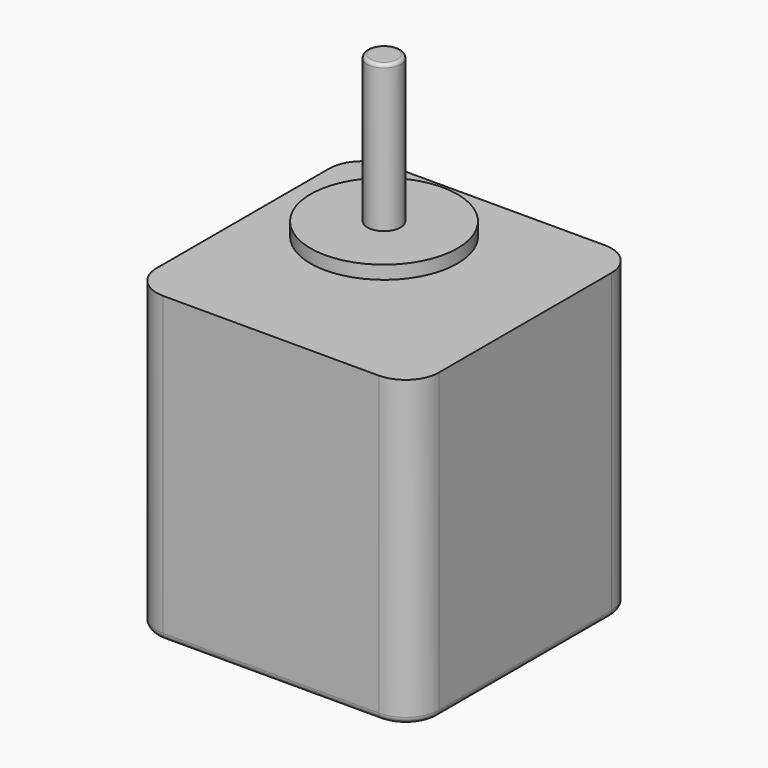
from build123d import *

# Parameters (mm, degrees)
F1_W     = 42.3
F1_H     = 42.3
F1_R     = 1.5
F1_R_2   = 11
F1_R_3   = 2.5
F2_DEPTH = 45.5
F3_START = 50
F3_DEPTH = 2
F4_START = 52
F4_DEPTH = 22
F5_R     = 0.5
F6_R     = 5
F7_R     = 1


with BuildPart() as f2:
    # F1 (on Top) → F2 (new body)
    with BuildSketch(Plane.XY):
        Rectangle(F1_W, F1_H)
        with Locations((-15.5, -15.5)):
            Circle(F1_R, mode=Mode.SUBTRACT)
        with Locations((15.5, -15.5)):
            Circle(F1_R, mode=Mode.SUBTRACT)
        with Locations((-15.5, 15.5)):
            Circle(F1_R, mode=Mode.SUBTRACT)
        Circle(F1_R_2, mode=Mode.SUBTRACT)
        with Locations((15.5, 15.5)):
            Circle(F1_R, mode=Mode.SUBTRACT)
        Circle(F1_R_2)
        Circle(F1_R_3, mode=Mode.SUBTRACT)
        Circle(F1_R_3)
        with Locations((-15.5, 15.5)):
            Circle(F1_R)
        with Locations((-15.5, -15.5)):
            Circle(F1_R)
        with Locations((15.5, -15.5)):
            Circle(F1_R)
        with Locations((15.5, 15.5)):
            Circle(F1_R)
    extrude(amount=F2_DEPTH)

    # F6
    f6_edges = [f2.edges().sort_by_distance(p)[0] for p in [
        (21.15, 21.15, 22.75),
        (-21.15, 21.15, 22.75),
        (-21.15, -21.15, 22.75),
        (21.15, -21.15, 22.75),
    ]]
    fillet(f6_edges, radius=F6_R)

    # F7
    f7_edges = [f2.edges().sort_by_distance(p)[0] for p in [
        (0, 21.15, 0),
        (19.685534, 19.685534, 0),
        (-19.685534, 19.685534, 0),
        (21.15, 0, 0),
        (-21.15, 0, 0),
        (19.685534, -19.685534, 0),
        (-19.685534, -19.685534, 0),
        (0, -21.15, 0),
    ]]
    fillet(f7_edges, radius=F7_R)


with BuildPart() as f3:
    # F1 (on Top) → F3 (new body)
    with BuildSketch(Plane.XY.offset(F3_START)):
        Circle(F1_R_2)
        Circle(F1_R_3, mode=Mode.SUBTRACT)
        Circle(F1_R_3)
    extrude(amount=F3_DEPTH)


with BuildPart() as f4:
    # F1 (on Top) → F4 (new body)
    with BuildSketch(Plane.XY.offset(F4_START)):
        Circle(F1_R_3)
    extrude(amount=F4_DEPTH)

    # F5
    f5_edges = [f4.edges().sort_by_distance(p)[0] for p in [
        (-2.5, 0, 74),
    ]]
    fillet(f5_edges, radius=F5_R)


solid = Compound([f2.part, f3.part, f4.part])
